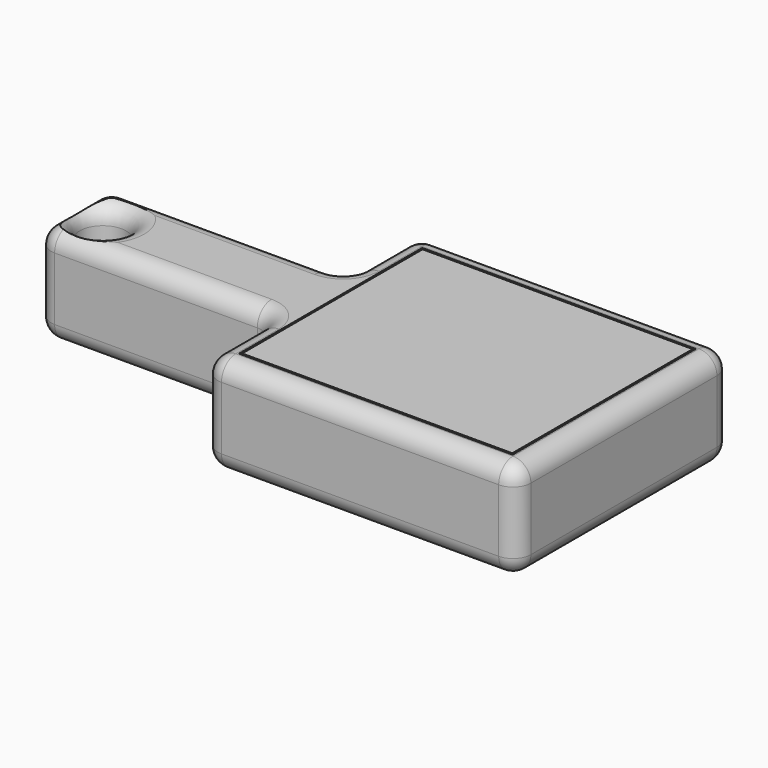
from build123d import *

# Parameters (mm, degrees)
F0_W           = 105.7696826756
F0_H           = 28.0387941748
F1_DEPTH       = 25.4
F2_W           = 38.074536249
F2_H           = 28.0387941748
F5_DEPTH       = 25.4
F4_W           = 38.074536249
F4_H           = 28.0387941748
F6_DEPTH       = 25.4
F7_DEPTH       = 50.8
F8_R           = 6.5972484206
F9_DEPTH       = 28.0397941748
F10_T1_DEPTH   = 28.0387941748
F10_T3_DEPTH   = 50.8
F10_T5_DEPTH   = 53.4387941748
F10_T7_DEPTH   = 96.494536249
F10_T9_DEPTH   = 17.8787941748
F10_T11_DEPTH  = 66.04
F10_S15_W      = 5.08
F10_S15_H      = 5.08
F10_T16_DEPTH  = 5.08
F10_S21_W      = 5.08
F10_S21_H      = 5.08
F10_T22_DEPTH  = 5.08
F10_S27_W      = 5.08
F10_S27_H      = 5.08
F10_T28_DEPTH  = 5.08
F10_S33_W      = 5.08
F10_S33_H      = 5.08
F10_T34_DEPTH  = 5.08
F10_T41_DEPTH  = 57.5351464266
F10_T43_DEPTH  = 15.24
F10_T45_DEPTH  = 15.24
F10_S49_W      = 5.08
F10_S49_H      = 5.08
F10_T50_DEPTH  = 5.08
F10_S55_W      = 5.08
F10_S55_H      = 5.08
F10_T56_DEPTH  = 5.08
F10_S61_W      = 5.08
F10_S61_H      = 5.08
F10_T62_DEPTH  = 5.08
F10_S67_W      = 5.08
F10_S67_H      = 5.08
F10_T68_DEPTH  = 5.08
F10_S73_W      = 5.08
F10_S73_H      = 5.08
F10_T74_DEPTH  = 5.08
F10_S79_W      = 5.08
F10_S79_H      = 5.08
F10_T80_DEPTH  = 5.08
F10_S85_W      = 5.08
F10_S85_H      = 5.08
F10_T86_DEPTH  = 5.08
F10_S91_W      = 5.08
F10_S91_H      = 5.08
F10_T92_DEPTH  = 5.08
F10_T96_ANGLE  = 90
F10_T98_ANGLE  = 90
F10_T100_ANGLE = 90
F10_T102_ANGLE = 90
F12_DEPTH      = 2.54


# Not quite as in the source:
# - a fillet or chamfer that OpenCascade refuses, or shapes differently, is made with other operations: its cross-section is extruded or revolved along the edge and cut away or added


with BuildPart() as f1:
    # F0 (on Front) → F1 (new body)
    with BuildSketch(Plane.XZ):
        with Locations((5.6814979762, 14.0193970874)):
            Rectangle(F0_W, F0_H)
    extrude(amount=F1_DEPTH)

    # F2 (on face) → F5 (join)
    with BuildSketch(Plane.XZ.offset(25.4)):
        with Locations((39.5290711895, 14.0193970874)):
            Rectangle(F2_W, F2_H)
    extrude(amount=F5_DEPTH)

    # F4 (on face) → F6 (join)
    with BuildSketch(Plane(origin=(0, 0, 0), x_dir=(-1, 0, 0), z_dir=(0, 1, 0))):
        with Locations((-39.5290711895, 14.0193970874)):
            Rectangle(F4_W, F4_H)
    extrude(amount=F6_DEPTH)

    # F7 (add): a face of the model
    f7_faces = [f1.faces().sort_by_distance(p)[0] for p in [
        (58.566339314, -12.7, 14.0193970874),
    ]]
    extrude(f7_faces, amount=F7_DEPTH)

    # F8 (on face) → F9 (cut, through all)
    with BuildSketch(Plane.XY.offset(28.0387941748)):
        with Locations((-37.849932909, -13.6290360242)):
            Circle(F8_R)
    extrude(amount=-F9_DEPTH, mode=Mode.SUBTRACT)

    # F10: fillet of radius 5.08 on 27 edges, made by hand

    # F10_s2 → F10_t1 (join)
    with BuildSketch(Plane.XY):
        with BuildLine():
            ThreePointArc((20.4918030649, -30.48), (19.0039055134, -26.8878975516), (15.4118030649, -25.4))
            Line((15.4118030649, -25.4), (20.4918030649, -25.4))
            Line((20.4918030649, -25.4), (20.4918030649, -30.48))
        make_face()
        with BuildLine():
            ThreePointArc((20.4918030649, 5.08), (19.0039055134, 1.4878975516), (15.4118030649, 0))
            Line((15.4118030649, 0), (20.4918030649, 0))
            Line((20.4918030649, 0), (20.4918030649, 5.08))
        make_face()
    extrude(amount=F10_T1_DEPTH)

    # F10_s4 → F10_t3 (cut)
    with BuildSketch(Plane.XZ.offset(-12.7)):
        with BuildLine():
            ThreePointArc((-42.1233433616, 28.0387941748), (-45.71544581, 26.5508966232), (-47.2033433616, 22.9587941748))
            Line((-47.2033433616, 22.9587941748), (-47.2033433616, 28.0387941748))
            Line((-47.2033433616, 28.0387941748), (-42.1233433616, 28.0387941748))
        make_face()
        with BuildLine():
            ThreePointArc((-47.2033433616, 5.08), (-45.71544581, 1.4878975516), (-42.1233433616, 0))
            Line((-42.1233433616, 0), (-47.2033433616, 0))
            Line((-47.2033433616, 0), (-47.2033433616, 5.08))
        make_face()
    extrude(amount=F10_T3_DEPTH, mode=Mode.SUBTRACT)

    # F10_s6 → F10_t5 (cut)
    with BuildSketch(Plane.XY.offset(-12.7)):
        with BuildLine():
            ThreePointArc((-47.2033433616, -5.08), (-45.71544581, -1.4878975516), (-42.1233433616, 0))
            Line((-42.1233433616, 0), (-47.2033433616, 0))
            Line((-47.2033433616, 0), (-47.2033433616, -5.08))
        make_face()
        with BuildLine():
            ThreePointArc((-42.1233433616, -25.4), (-45.71544581, -23.9121024484), (-47.2033433616, -20.32))
            Line((-47.2033433616, -20.32), (-47.2033433616, -25.4))
            Line((-47.2033433616, -25.4), (-42.1233433616, -25.4))
        make_face()
        with BuildLine():
            ThreePointArc((25.5718030649, 25.4), (21.9797006165, 23.9121024484), (20.4918030649, 20.32))
            Line((20.4918030649, 20.32), (20.4918030649, 25.4))
            Line((20.4918030649, 25.4), (25.5718030649, 25.4))
        make_face()
        with BuildLine():
            ThreePointArc((25.5718030649, -50.8), (21.9797006165, -49.3121024484), (20.4918030649, -45.72))
            Line((20.4918030649, -45.72), (20.4918030649, -50.8))
            Line((20.4918030649, -50.8), (25.5718030649, -50.8))
        make_face()
    extrude(amount=F10_T5_DEPTH, mode=Mode.SUBTRACT)

    # F10_s8 → F10_t7 (cut)
    with BuildSketch(Plane.YZ.offset(7.7918030649)):
        with BuildLine():
            ThreePointArc((-50.8, 5.08), (-49.3121024484, 1.4878975516), (-45.72, 0))
            Line((-45.72, 0), (-50.8, 0))
            Line((-50.8, 0), (-50.8, 5.08))
        make_face()
        with BuildLine():
            ThreePointArc((-45.72, 28.0387941748), (-49.3121024484, 26.5508966232), (-50.8, 22.9587941748))
            Line((-50.8, 22.9587941748), (-50.8, 28.0387941748))
            Line((-50.8, 28.0387941748), (-45.72, 28.0387941748))
        make_face()
        with BuildLine():
            ThreePointArc((25.4, 5.08), (23.9121024484, 1.4878975516), (20.32, 0))
            Line((20.32, 0), (25.4, 0))
            Line((25.4, 0), (25.4, 5.08))
        make_face()
        with BuildLine():
            ThreePointArc((20.32, 28.0387941748), (23.9121024484, 26.5508966232), (25.4, 22.9587941748))
            Line((25.4, 22.9587941748), (25.4, 28.0387941748))
            Line((25.4, 28.0387941748), (20.32, 28.0387941748))
        make_face()
    extrude(amount=F10_T7_DEPTH, mode=Mode.SUBTRACT)

    # F10_s10 → F10_t9 (cut)
    with BuildSketch(Plane.XY.offset(5.08)):
        with BuildLine():
            ThreePointArc((104.286339314, -50.8), (107.8784417624, -49.3121024484), (109.366339314, -45.72))
            Line((109.366339314, -45.72), (109.366339314, -50.8))
            Line((109.366339314, -50.8), (104.286339314, -50.8))
        make_face()
        with BuildLine():
            ThreePointArc((109.366339314, 20.32), (107.8784417624, 23.9121024484), (104.286339314, 25.4))
            Line((104.286339314, 25.4), (109.366339314, 25.4))
            Line((109.366339314, 25.4), (109.366339314, 20.32))
        make_face()
    extrude(amount=F10_T9_DEPTH, mode=Mode.SUBTRACT)

    # F10_s12 → F10_t11 (cut)
    with BuildSketch(Plane.XZ.offset(-20.32)):
        with BuildLine():
            ThreePointArc((109.366339314, 5.08), (107.8784417624, 1.4878975516), (104.286339314, 0))
            Line((104.286339314, 0), (109.366339314, 0))
            Line((109.366339314, 0), (109.366339314, 5.08))
        make_face()
        with BuildLine():
            ThreePointArc((104.286339314, 28.0387941748), (107.8784417624, 26.5508966232), (109.366339314, 22.9587941748))
            Line((109.366339314, 22.9587941748), (109.366339314, 28.0387941748))
            Line((109.366339314, 28.0387941748), (104.286339314, 28.0387941748))
        make_face()
    extrude(amount=F10_T11_DEPTH, mode=Mode.SUBTRACT)


with BuildPart() as f10_tool14:
    # F10_s15 → F10_t16 (new body)
    with BuildSketch(Plane.XZ.offset(45.72)):
        with Locations((106.826339314, 2.54)):
            Rectangle(F10_S15_W, F10_S15_H)
    extrude(amount=F10_T16_DEPTH)

    # F10_s17 → F10_t18 (revolve, cut)
    with BuildSketch(Plane(origin=(104.286339314, -45.72, 5.08), x_dir=(-0.7071067812, 0, 0.7071067812), z_dir=(0.7071067812, 0, 0.7071067812))):
        with BuildLine():
            ThreePointArc((0, -5.08), (5.08, 0), (0, 5.08))
            Line((0, 5.08), (0, -5.08))
        make_face()
    revolve(axis=Axis((104.286339314, -45.72, 5.08), (0, -1, 0)), mode=Mode.SUBTRACT)


with BuildPart() as f1_1:
    add(f1.part)

    # F10_t13: cut F10_tool14
    add(f10_tool14.part, mode=Mode.SUBTRACT)


with BuildPart() as f10_tool20:
    # F10_s21 → F10_t22 (new body)
    with BuildSketch(Plane.XY.offset(22.9587941748)):
        with Locations((106.826339314, -48.26)):
            Rectangle(F10_S21_W, F10_S21_H)
    extrude(amount=F10_T22_DEPTH)

    # F10_s23 → F10_t24 (revolve, cut)
    with BuildSketch(Plane(origin=(104.286339314, -45.72, 22.9587941748), x_dir=(-0.7071067812, 0.7071067812, 0), z_dir=(0.7071067812, 0.7071067812, 0))):
        with BuildLine():
            ThreePointArc((0, -5.08), (5.08, 0), (0, 5.08))
            Line((0, 5.08), (0, -5.08))
        make_face()
    revolve(axis=Axis((104.286339314, -45.72, 22.9587941748), (0, 0, 1)), mode=Mode.SUBTRACT)


with BuildPart() as f1_2:
    add(f1_1.part)

    # F10_t19: cut F10_tool20
    add(f10_tool20.part, mode=Mode.SUBTRACT)


with BuildPart() as f10_tool26:
    # F10_s27 → F10_t28 (new body)
    with BuildSketch(Plane.XY.offset(5.08)):
        with Locations((106.826339314, 22.86)):
            Rectangle(F10_S27_W, F10_S27_H)
    extrude(amount=-F10_T28_DEPTH)

    # F10_s29 → F10_t30 (revolve, cut)
    with BuildSketch(Plane(origin=(104.286339314, 20.32, 5.08), x_dir=(-0.7071067812, -0.7071067812, 0), z_dir=(0.7071067812, -0.7071067812, 0))):
        with BuildLine():
            ThreePointArc((0, -5.08), (5.08, 0), (0, 5.08))
            Line((0, 5.08), (0, -5.08))
        make_face()
    revolve(axis=Axis((104.286339314, 20.32, 5.08), (0, 0, -1)), mode=Mode.SUBTRACT)


with BuildPart() as f1_3:
    add(f1_2.part)

    # F10_t25: cut F10_tool26
    add(f10_tool26.part, mode=Mode.SUBTRACT)


with BuildPart() as f10_tool32:
    # F10_s33 → F10_t34 (new body)
    with BuildSketch(Plane.XY.offset(22.9587941748)):
        with Locations((106.826339314, 22.86)):
            Rectangle(F10_S33_W, F10_S33_H)
    extrude(amount=F10_T34_DEPTH)

    # F10_s35 → F10_t36 (revolve, cut)
    with BuildSketch(Plane(origin=(104.286339314, 20.32, 22.9587941748), x_dir=(-0.7071067812, -0.7071067812, 0), z_dir=(-0.7071067812, 0.7071067812, 0))):
        with BuildLine():
            ThreePointArc((0, -5.08), (5.08, 0), (0, 5.08))
            Line((0, 5.08), (0, -5.08))
        make_face()
    revolve(axis=Axis((104.286339314, 20.32, 22.9587941748), (0, 0, 1)), mode=Mode.SUBTRACT)


with BuildPart() as f1_4:
    add(f1_3.part)

    # F10_t31: cut F10_tool32
    add(f10_tool32.part, mode=Mode.SUBTRACT)

    # F10_s37 → F10_t38 (revolve, cut)
    with BuildSketch(Plane.XZ.offset(13.6290360242)):
        with BuildLine():
            ThreePointArc((-26.1726844884, 28.0387941748), (-29.7647869368, 26.5508966232), (-31.2526844884, 22.9587941748))
            Line((-31.2526844884, 22.9587941748), (-31.2526844884, 28.0387941748))
            Line((-31.2526844884, 28.0387941748), (-26.1726844884, 28.0387941748))
        make_face()
    revolve(axis=Axis((-37.849932909, -13.6290360242, 28.0387941748), (0, 0, 1)), mode=Mode.SUBTRACT)

    # F10_s39 → F10_t40 (revolve, cut)
    with BuildSketch(Plane.XZ.offset(13.6290360242)):
        with BuildLine():
            ThreePointArc((-31.2526844884, 5.08), (-29.7647869368, 1.4878975516), (-26.1726844884, 0))
            Line((-26.1726844884, 0), (-31.2526844884, 0))
            Line((-31.2526844884, 0), (-31.2526844884, 5.08))
        make_face()
    revolve(axis=Axis((-37.849932909, -13.6290360242, 0), (0, 0, 1)), mode=Mode.SUBTRACT)

    # F10_s42 → F10_t41 (cut)
    with BuildSketch(Plane.YZ.offset(-42.1233433616)):
        with BuildLine():
            ThreePointArc((-5.08, 28.0387941748), (-1.4878975516, 26.5508966232), (0, 22.9587941748))
            Line((0, 22.9587941748), (0, 28.0387941748))
            Line((0, 28.0387941748), (-5.08, 28.0387941748))
        make_face()
        with BuildLine():
            ThreePointArc((-20.32, 28.0387941748), (-23.9121024484, 26.5508966232), (-25.4, 22.9587941748))
            Line((-25.4, 22.9587941748), (-25.4, 28.0387941748))
            Line((-25.4, 28.0387941748), (-20.32, 28.0387941748))
        make_face()
        with BuildLine():
            ThreePointArc((-25.4, 5.08), (-23.9121024484, 1.4878975516), (-20.32, 0))
            Line((-20.32, 0), (-25.4, 0))
            Line((-25.4, 0), (-25.4, 5.08))
        make_face()
        with BuildLine():
            ThreePointArc((0, 5.08), (-1.4878975516, 1.4878975516), (-5.08, 0))
            Line((-5.08, 0), (0, 0))
            Line((0, 0), (0, 5.08))
        make_face()
    extrude(amount=F10_T41_DEPTH, mode=Mode.SUBTRACT)

    # F10_s44 → F10_t43 (cut)
    with BuildSketch(Plane.XZ.offset(-20.32)):
        with BuildLine():
            ThreePointArc((20.4918030649, 5.08), (21.9797006165, 1.4878975516), (25.5718030649, 0))
            Line((25.5718030649, 0), (20.4918030649, 0))
            Line((20.4918030649, 0), (20.4918030649, 5.08))
        make_face()
        with BuildLine():
            ThreePointArc((25.5718030649, 28.0387941748), (21.9797006165, 26.5508966232), (20.4918030649, 22.9587941748))
            Line((20.4918030649, 22.9587941748), (20.4918030649, 28.0387941748))
            Line((20.4918030649, 28.0387941748), (25.5718030649, 28.0387941748))
        make_face()
    extrude(amount=F10_T43_DEPTH, mode=Mode.SUBTRACT)

    # F10_s46 → F10_t45 (cut)
    with BuildSketch(Plane.XZ.offset(30.48)):
        with BuildLine():
            ThreePointArc((20.4918030649, 5.08), (21.9797006165, 1.4878975516), (25.5718030649, 0))
            Line((25.5718030649, 0), (20.4918030649, 0))
            Line((20.4918030649, 0), (20.4918030649, 5.08))
        make_face()
        with BuildLine():
            ThreePointArc((25.5718030649, 28.0387941748), (21.9797006165, 26.5508966232), (20.4918030649, 22.9587941748))
            Line((20.4918030649, 22.9587941748), (20.4918030649, 28.0387941748))
            Line((20.4918030649, 28.0387941748), (25.5718030649, 28.0387941748))
        make_face()
    extrude(amount=F10_T45_DEPTH, mode=Mode.SUBTRACT)


with BuildPart() as f10_tool48:
    # F10_s49 → F10_t50 (new body)
    with BuildSketch(Plane.XZ.offset(5.08)):
        with Locations((-44.6633433616, 2.54)):
            Rectangle(F10_S49_W, F10_S49_H)
    extrude(amount=-F10_T50_DEPTH)

    # F10_s51 → F10_t52 (revolve, cut)
    with BuildSketch(Plane(origin=(-42.1233433616, -5.08, 5.08), x_dir=(0.7071067812, 0, 0.7071067812), z_dir=(-0.7071067812, 0, 0.7071067812))):
        with BuildLine():
            ThreePointArc((0, -5.08), (5.08, 0), (0, 5.08))
            Line((0, 5.08), (0, -5.08))
        make_face()
    revolve(axis=Axis((-42.1233433616, -5.08, 5.08), (0, 1, 0)), mode=Mode.SUBTRACT)


with BuildPart() as f1_5:
    add(f1_4.part)

    # F10_t47: cut F10_tool48
    add(f10_tool48.part, mode=Mode.SUBTRACT)


with BuildPart() as f10_tool54:
    # F10_s55 → F10_t56 (new body)
    with BuildSketch(Plane.XZ.offset(20.32)):
        with Locations((-44.6633433616, 2.54)):
            Rectangle(F10_S55_W, F10_S55_H)
    extrude(amount=F10_T56_DEPTH)

    # F10_s57 → F10_t58 (revolve, cut)
    with BuildSketch(Plane(origin=(-42.1233433616, -20.32, 5.08), x_dir=(0.7071067812, 0, 0.7071067812), z_dir=(0.7071067812, 0, -0.7071067812))):
        with BuildLine():
            ThreePointArc((0, -5.08), (5.08, 0), (0, 5.08))
            Line((0, 5.08), (0, -5.08))
        make_face()
    revolve(axis=Axis((-42.1233433616, -20.32, 5.08), (0, -1, 0)), mode=Mode.SUBTRACT)


with BuildPart() as f1_6:
    add(f1_5.part)

    # F10_t53: cut F10_tool54
    add(f10_tool54.part, mode=Mode.SUBTRACT)


with BuildPart() as f10_tool60:
    # F10_s61 → F10_t62 (new body)
    with BuildSketch(Plane.XY.offset(22.9587941748)):
        with Locations((23.0318030649, 22.86)):
            Rectangle(F10_S61_W, F10_S61_H)
    extrude(amount=F10_T62_DEPTH)

    # F10_s63 → F10_t64 (revolve, cut)
    with BuildSketch(Plane(origin=(25.5718030649, 20.32, 22.9587941748), x_dir=(0.7071067812, -0.7071067812, 0), z_dir=(-0.7071067812, -0.7071067812, 0))):
        with BuildLine():
            ThreePointArc((0, -5.08), (5.08, 0), (0, 5.08))
            Line((0, 5.08), (0, -5.08))
        make_face()
    revolve(axis=Axis((25.5718030649, 20.32, 22.9587941748), (0, 0, 1)), mode=Mode.SUBTRACT)


with BuildPart() as f1_7:
    add(f1_6.part)

    # F10_t59: cut F10_tool60
    add(f10_tool60.part, mode=Mode.SUBTRACT)


with BuildPart() as f10_tool66:
    # F10_s67 → F10_t68 (new body)
    with BuildSketch(Plane.XY.offset(22.9587941748)):
        with Locations((23.0318030649, -48.26)):
            Rectangle(F10_S67_W, F10_S67_H)
    extrude(amount=F10_T68_DEPTH)

    # F10_s69 → F10_t70 (revolve, cut)
    with BuildSketch(Plane(origin=(25.5718030649, -45.72, 22.9587941748), x_dir=(0.7071067812, 0.7071067812, 0), z_dir=(0.7071067812, -0.7071067812, 0))):
        with BuildLine():
            ThreePointArc((0, -5.08), (5.08, 0), (0, 5.08))
            Line((0, 5.08), (0, -5.08))
        make_face()
    revolve(axis=Axis((25.5718030649, -45.72, 22.9587941748), (0, 0, 1)), mode=Mode.SUBTRACT)


with BuildPart() as f1_8:
    add(f1_7.part)

    # F10_t65: cut F10_tool66
    add(f10_tool66.part, mode=Mode.SUBTRACT)


with BuildPart() as f10_tool72:
    # F10_s73 → F10_t74 (new body)
    with BuildSketch(Plane.YZ.offset(25.5718030649)):
        with Locations((-48.26, 2.54)):
            Rectangle(F10_S73_W, F10_S73_H)
    extrude(amount=-F10_T74_DEPTH)

    # F10_s75 → F10_t76 (revolve, cut)
    with BuildSketch(Plane(origin=(25.5718030649, -45.72, 5.08), x_dir=(0, 0.7071067812, 0.7071067812), z_dir=(0, -0.7071067812, 0.7071067812))):
        with BuildLine():
            ThreePointArc((0, -5.08), (5.08, 0), (0, 5.08))
            Line((0, 5.08), (0, -5.08))
        make_face()
    revolve(axis=Axis((25.5718030649, -45.72, 5.08), (-1, 0, 0)), mode=Mode.SUBTRACT)


with BuildPart() as f1_9:
    add(f1_8.part)

    # F10_t71: cut F10_tool72
    add(f10_tool72.part, mode=Mode.SUBTRACT)


with BuildPart() as f10_tool78:
    # F10_s79 → F10_t80 (new body)
    with BuildSketch(Plane.YZ.offset(25.5718030649)):
        with Locations((22.86, 2.54)):
            Rectangle(F10_S79_W, F10_S79_H)
    extrude(amount=-F10_T80_DEPTH)

    # F10_s81 → F10_t82 (revolve, cut)
    with BuildSketch(Plane(origin=(25.5718030649, 20.32, 5.08), x_dir=(0, -0.7071067812, 0.7071067812), z_dir=(0, -0.7071067812, -0.7071067812))):
        with BuildLine():
            ThreePointArc((0, -5.08), (5.08, 0), (0, 5.08))
            Line((0, 5.08), (0, -5.08))
        make_face()
    revolve(axis=Axis((25.5718030649, 20.32, 5.08), (-1, 0, 0)), mode=Mode.SUBTRACT)


with BuildPart() as f1_10:
    add(f1_9.part)

    # F10_t77: cut F10_tool78
    add(f10_tool78.part, mode=Mode.SUBTRACT)


with BuildPart() as f10_tool84:
    # F10_s85 → F10_t86 (new body)
    with BuildSketch(Plane.XY.offset(22.9587941748)):
        with Locations((-44.6633433616, -22.86)):
            Rectangle(F10_S85_W, F10_S85_H)
    extrude(amount=F10_T86_DEPTH)

    # F10_s87 → F10_t88 (revolve, cut)
    with BuildSketch(Plane(origin=(-42.1233433616, -20.32, 22.9587941748), x_dir=(0.7071067812, 0.7071067812, 0), z_dir=(0.7071067812, -0.7071067812, 0))):
        with BuildLine():
            ThreePointArc((0, -5.08), (5.08, 0), (0, 5.08))
            Line((0, 5.08), (0, -5.08))
        make_face()
    revolve(axis=Axis((-42.1233433616, -20.32, 22.9587941748), (0, 0, 1)), mode=Mode.SUBTRACT)


with BuildPart() as f1_11:
    add(f1_10.part)

    # F10_t83: cut F10_tool84
    add(f10_tool84.part, mode=Mode.SUBTRACT)


with BuildPart() as f10_tool90:
    # F10_s91 → F10_t92 (new body)
    with BuildSketch(Plane.XY.offset(22.9587941748)):
        with Locations((-44.6633433616, -2.54)):
            Rectangle(F10_S91_W, F10_S91_H)
    extrude(amount=F10_T92_DEPTH)

    # F10_s93 → F10_t94 (revolve, cut)
    with BuildSketch(Plane(origin=(-42.1233433616, -5.08, 22.9587941748), x_dir=(0.7071067812, -0.7071067812, 0), z_dir=(-0.7071067812, -0.7071067812, 0))):
        with BuildLine():
            ThreePointArc((0, -5.08), (5.08, 0), (0, 5.08))
            Line((0, 5.08), (0, -5.08))
        make_face()
    revolve(axis=Axis((-42.1233433616, -5.08, 22.9587941748), (0, 0, 1)), mode=Mode.SUBTRACT)


with BuildPart() as f1_12:
    add(f1_11.part)

    # F10_t89: cut F10_tool90
    add(f10_tool90.part, mode=Mode.SUBTRACT)

    # F10_s95 → F10_t96 (revolve, cut)
    with BuildSketch(Plane.XZ.offset(-5.08)):
        with BuildLine():
            ThreePointArc((20.4918030649, 5.08), (21.9797006165, 1.4878975516), (25.5718030649, 0))
            Line((25.5718030649, 0), (20.4918030649, 0))
            Line((20.4918030649, 0), (20.4918030649, 5.08))
        make_face()
    revolve(axis=Axis((15.4118030649, 5.08, 0), (0, 0, -1)), revolution_arc=F10_T96_ANGLE, mode=Mode.SUBTRACT)

    # F10_s97 → F10_t98 (revolve, cut)
    with BuildSketch(Plane.XZ.offset(30.48)):
        with BuildLine():
            ThreePointArc((20.4918030649, 5.08), (21.9797006165, 1.4878975516), (25.5718030649, 0))
            Line((25.5718030649, 0), (20.4918030649, 0))
            Line((20.4918030649, 0), (20.4918030649, 5.08))
        make_face()
    revolve(axis=Axis((15.4118030649, -30.48, 0), (0, 0, 1)), revolution_arc=F10_T98_ANGLE, mode=Mode.SUBTRACT)

    # F10_s99 → F10_t100 (revolve, cut)
    with BuildSketch(Plane.XZ.offset(-5.08)):
        with BuildLine():
            ThreePointArc((25.5718030649, 28.0387941748), (21.9797006165, 26.5508966232), (20.4918030649, 22.9587941748))
            Line((20.4918030649, 22.9587941748), (20.4918030649, 28.0387941748))
            Line((20.4918030649, 28.0387941748), (25.5718030649, 28.0387941748))
        make_face()
    revolve(axis=Axis((15.4118030649, 5.08, 28.0387941748), (0, 0, -1)), revolution_arc=F10_T100_ANGLE, mode=Mode.SUBTRACT)

    # F10_s101 → F10_t102 (revolve, cut)
    with BuildSketch(Plane.XZ.offset(30.48)):
        with BuildLine():
            ThreePointArc((25.5718030649, 28.0387941748), (21.9797006165, 26.5508966232), (20.4918030649, 22.9587941748))
            Line((20.4918030649, 22.9587941748), (20.4918030649, 28.0387941748))
            Line((20.4918030649, 28.0387941748), (25.5718030649, 28.0387941748))
        make_face()
    revolve(axis=Axis((15.4118030649, -30.48, 28.0387941748), (0, 0, 1)), revolution_arc=F10_T102_ANGLE, mode=Mode.SUBTRACT)

    # F11 (on face) → F12 (cut)
    with BuildSketch(Plane.XY.offset(28.0387941748)):
        Polygon((103.778339314, -45.212), (103.778339314, 19.812), (26.0798030649, 19.812), (26.0798030649, -30.48), (26.0798030649, -45.212), align=None)
        Polygon((26.5878030649, -44.704), (26.5878030649, -30.48), (26.5878030649, 19.304), (103.270339314, 19.304), (103.270339314, -44.704), align=None, mode=Mode.SUBTRACT)
    extrude(amount=-F12_DEPTH, mode=Mode.SUBTRACT)


solid = f1_12.part
